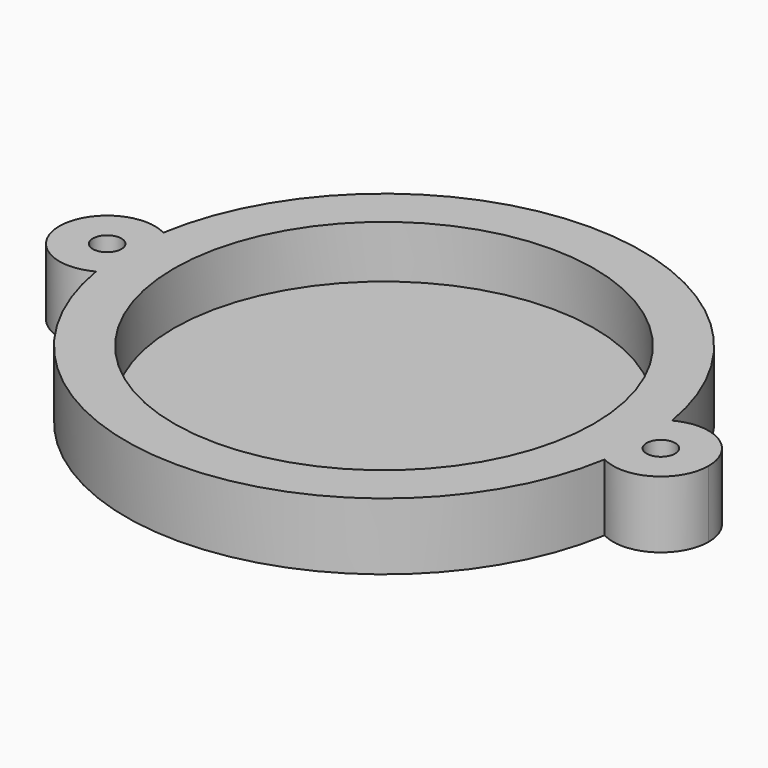
from build123d import *

# Parameters (mm, degrees)
F0_R     = 1.5
F1_DEPTH = 7
F2_DEPTH = 7
F3_R     = 22
F4_DEPTH = 5.5


with BuildPart() as f1:
    # F0 (on Top) → F1 (new body)
    with BuildSketch(Plane.XY):
        with BuildLine():
            ThreePointArc((-26.6379310345, -4.4068844099), (-27, 0), (-26.6379310345, 4.4068844099))
            ThreePointArc((-26.6379310345, 4.4068844099), (-34, 0), (-26.6379310345, -4.4068844099))
        make_face()
        with Locations((-29, 0)):
            Circle(F0_R, mode=Mode.SUBTRACT)
    extrude(amount=F1_DEPTH)



with BuildPart() as f1b:
    # F0 (on Top) → F1, piece 2 (new body)
    with BuildSketch(Plane.XY):
        with BuildLine():
            ThreePointArc((26.6379310345, 4.4068844099), (26.9093305187, 2.21086658), (27, 0))
            ThreePointArc((27, 0), (26.9093305187, -2.21086658), (26.6379310345, -4.4068844099))
            ThreePointArc((26.6379310345, -4.4068844099), (31.5680396388, -4.2901249881), (34, 0))
            ThreePointArc((34, 0), (31.5680396388, 4.2901249881), (26.6379310345, 4.4068844099))
        make_face()
        with Locations((29, 0)):
            Circle(F0_R, mode=Mode.SUBTRACT)
    extrude(amount=F1_DEPTH)


with BuildPart() as f1_1:
    add(f1.part)

    add(f1b.part)  # F2 merges F1b
    # F0 (on Top) → F2 (join)
    with BuildSketch(Plane.XY):
        with BuildLine():
            ThreePointArc((-24, 0), (-24.7098750119, 2.5680396388), (-26.6379310345, 4.4068844099))
            ThreePointArc((-26.6379310345, 4.4068844099), (-27, 0), (-26.6379310345, -4.4068844099))
            ThreePointArc((-26.6379310345, -4.4068844099), (-24.7098750119, -2.5680396388), (-24, 0))
        make_face()
        with BuildLine():
            ThreePointArc((26.6379310345, -4.4068844099), (26.9093305187, -2.21086658), (27, 0))
            ThreePointArc((27, 0), (26.9093305187, 2.21086658), (26.6379310345, 4.4068844099))
            ThreePointArc((26.6379310345, 4.4068844099), (24, 0), (26.6379310345, -4.4068844099))
        make_face()
        with BuildLine():
            ThreePointArc((26.6379310345, -4.4068844099), (24, 0), (26.6379310345, 4.4068844099))
            ThreePointArc((26.6379310345, 4.4068844099), (0, 27), (-26.6379310345, 4.4068844099))
            ThreePointArc((-26.6379310345, 4.4068844099), (-24.7098750119, 2.5680396388), (-24, 0))
            ThreePointArc((-24, 0), (-24.7098750119, -2.5680396388), (-26.6379310345, -4.4068844099))
            ThreePointArc((-26.6379310345, -4.4068844099), (0, -27), (26.6379310345, -4.4068844099))
        make_face()
    extrude(amount=F2_DEPTH)

    # F3 (on face) → F4 (cut)
    with BuildSketch(Plane.XY.offset(7)):
        Circle(F3_R)
    extrude(amount=-F4_DEPTH, mode=Mode.SUBTRACT)


solid = f1_1.part
